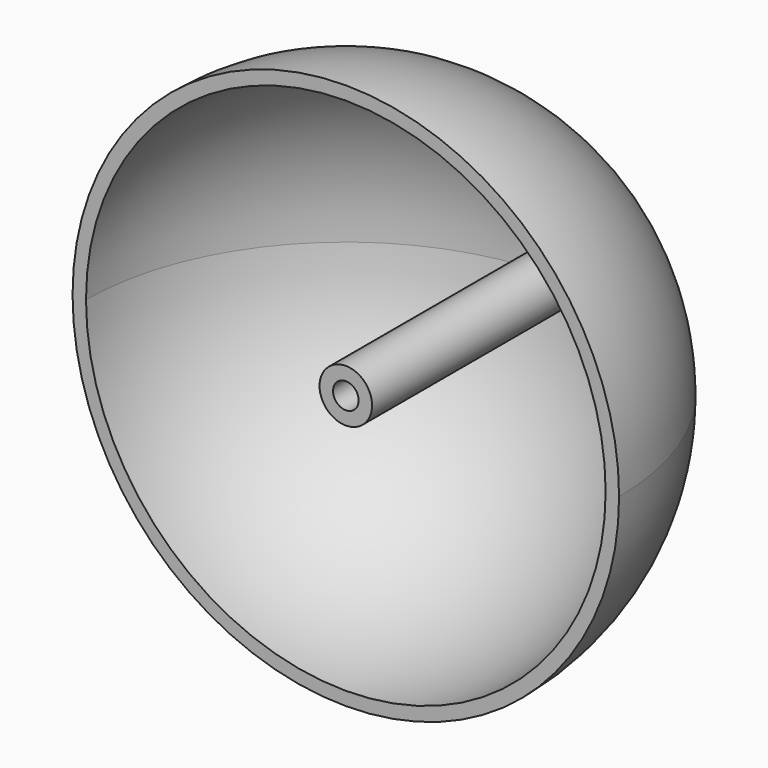
from build123d import *

# Parameters (mm, degrees)
F1_ANGLE = 180
F2_D     = 4.7625
F4_T     = -2.5


# Not quite as in the source:
# - a feature of the source that left no trace in its solid (it failed there, or was rolled back) is left out


with BuildPart() as f1:
    # F0 (on Front) → F1 (revolve)
    with BuildSketch(Plane.XZ):
        with BuildLine():
            ThreePointArc((0, -50.8), (35.9210244843, -35.9210244843), (50.8, 0))
            ThreePointArc((50.8, 0), (35.9210244843, 35.9210244843), (0, 50.8))
            Line((0, 50.8), (0, 0))
            Line((0, 0), (0, -50.8))
        make_face()
    revolve(axis=Axis((0, 0, 25.4), (0, 0, 1)), revolution_arc=F1_ANGLE)

    # F2 (through all)
    with Locations(Plane.XZ):
        with Locations((0, 0)):
            Hole(F2_D / 2)

    # F4
    f4_openings = [f1.faces().sort_by_distance(p)[0] for p in [
        (49.363159, 0, 0),
    ]]
    offset(amount=F4_T, openings=f4_openings)


solid = f1.part
